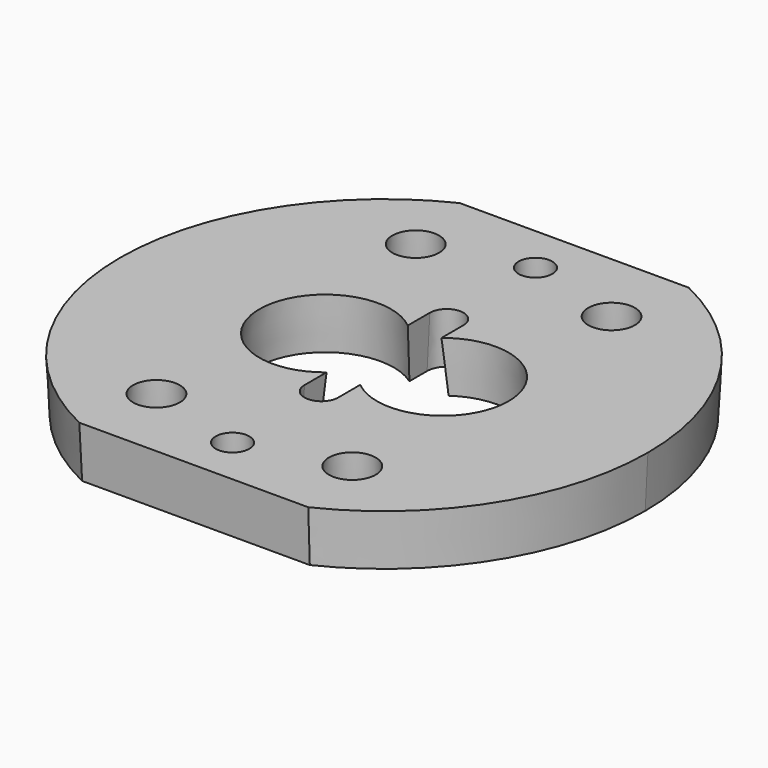
from build123d import *

# Parameters (mm, degrees)
F0_R                   = 2
F0_R_2                 = 1.5
F1_DEPTH               = 4
DRAFT_F1_DRAFTED_ANGLE = -3


# Not quite as in the source:
# - an extrude with a draft is written as a straight extrude whose walls are then drafted


with BuildPart() as f1:
    # F0 (on Top) → F1 (new body)
    with BuildSketch(Plane.XY):
        with BuildLine():
            ThreePointArc((8.7177978871, -18), (16.9463264123, -10.6217710919), (20, 0))
            ThreePointArc((20, 0), (16.9463264123, 10.6217710919), (8.7177978871, 18))
            Line((8.7177978871, 18), (-8.7177978871, 18))
            ThreePointArc((-8.7177978871, 18), (-20, 0), (-8.7177978871, -18))
            Line((-8.7177978871, -18), (8.7177978871, -18))
        make_face()
        with Locations((-7.5, -12.409673646)):
            Circle(F0_R, mode=Mode.SUBTRACT)
        with Locations((0, -14.5)):
            Circle(F0_R_2, mode=Mode.SUBTRACT)
        with Locations((7.5, -12.409673646)):
            Circle(F0_R, mode=Mode.SUBTRACT)
        with Locations((-7.5, 12.409673646)):
            Circle(F0_R, mode=Mode.SUBTRACT)
        with BuildLine():
            ThreePointArc((1.5, 4.3084219849), (6.9302777619, 4.6536276172), (9.75, 0))
            ThreePointArc((9.75, 0), (6.9302777619, -4.6536276172), (1.5, -4.3084219849))
            Line((1.5, -4.3084219849), (1.5, -6))
            ThreePointArc((1.5, -6), (0, -7.5), (-1.5, -6))
            Line((-1.5, -6), (-1.5, -4.3084219849))
            ThreePointArc((-1.5, -4.3084219849), (-9.75, 0), (-1.5, 4.3084219849))
            Line((-1.5, 4.3084219849), (-1.5, 6))
            ThreePointArc((-1.5, 6), (0, 7.5), (1.5, 6))
            Line((1.5, 6), (1.5, 4.3084219849))
        make_face(mode=Mode.SUBTRACT)
        with Locations((0, 14.5)):
            Circle(F0_R_2, mode=Mode.SUBTRACT)
        with Locations((7.5, 12.409673646)):
            Circle(F0_R, mode=Mode.SUBTRACT)
    extrude(amount=F1_DEPTH)

    # draft_F1_drafted
    draft_f1_drafted_walls = [f1.faces().sort_by_distance(p)[0] for p in [
        (0, -18, 2.6666666667),
        (5.5, 12.409673646, 2.6666666667),
        (-1.5, 14.5, 2.6666666667),
        (1.5, 5.1542109925, 2.6666666667),
        (0, 7.5, 2.6666666667),
        (-1.5, 5.1542109925, 2.6666666667),
        (-9.75, 0, 2.6666666667),
        (-1.5, -5.1542109925, 2.6666666667),
        (0, -7.5, 2.6666666667),
        (1.5, -5.1542109925, 2.6666666667),
        (9.75, 0, 2.6666666667),
        (-9.5, 12.409673646, 2.6666666667),
        (5.5, -12.409673646, 2.6666666667),
        (-1.5, -14.5, 2.6666666667),
        (-9.5, -12.409673646, 2.6666666667),
        (0, 18, 2.6666666667),
        (20, 0, 2.6666666667),
        (-20, 0, 2.6666666667),
    ]]
    draft(draft_f1_drafted_walls, neutral_plane=Plane.XY, angle=DRAFT_F1_DRAFTED_ANGLE)


solid = f1.part
